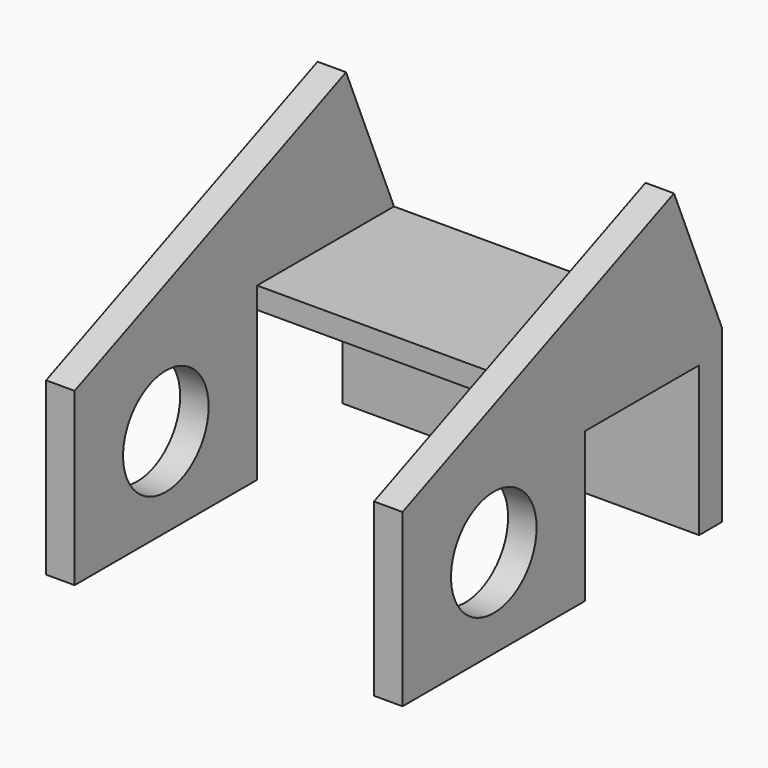
from build123d import *

# Parameters (mm, degrees)
F0_W     = 63.5
F0_H     = 30.48
F1_DEPTH = 71.12
F2_W     = 53.34
F2_H     = 30.48
F3_DEPTH = 40.64
F4_R     = 9.525
F4_W     = 25.4
F4_H     = 26.6478173435
F5_DEPTH = 63.5
F7_DEPTH = 5.08
F9_DEPTH = 5.08


# Not quite as in the source:
# - a feature names something its author has since deleted; it is built from what else it names


with BuildPart() as f1:
    # F0 (on Front) → F1 (new body)
    with BuildSketch(Plane.XZ):
        with Locations((31.75, 15.24)):
            Rectangle(F0_W, F0_H)
    extrude(amount=F1_DEPTH)

    # F2 (on face) → F3 (cut)
    with BuildSketch(Plane.XZ.offset(71.12)):
        with Locations((31.75, 15.24)):
            Rectangle(F2_W, F2_H)
    extrude(amount=-F3_DEPTH, mode=Mode.SUBTRACT)

    # F4 (on face) → F5 (cut)
    with BuildSketch(Plane.YZ.offset(63.5)):
        with Locations((-50.8, 15.8844571561)):
            Circle(F4_R)
        with Locations((-17.78, 13.3239086717)):
            Rectangle(F4_W, F4_H)
    extrude(amount=-F5_DEPTH, mode=Mode.SUBTRACT)

    # F6 (on face) → F7 (join)
    with BuildSketch(Plane.YZ.offset(63.5)):
        Polygon((-10.6731842133, 55.88), (-71.12, 30.48), (0, 30.48), align=None)
    extrude(amount=-F7_DEPTH)

    # F8 (on face) → F9 (join)
    with BuildSketch(Plane(origin=(0, 0, 0), x_dir=(0, -1, 0), z_dir=(-1, 0, 0))):
        Polygon((10.6731842133, 55.88), (0, 30.48), (71.12, 30.48), align=None)
    extrude(amount=-F9_DEPTH)


solid = f1.part
